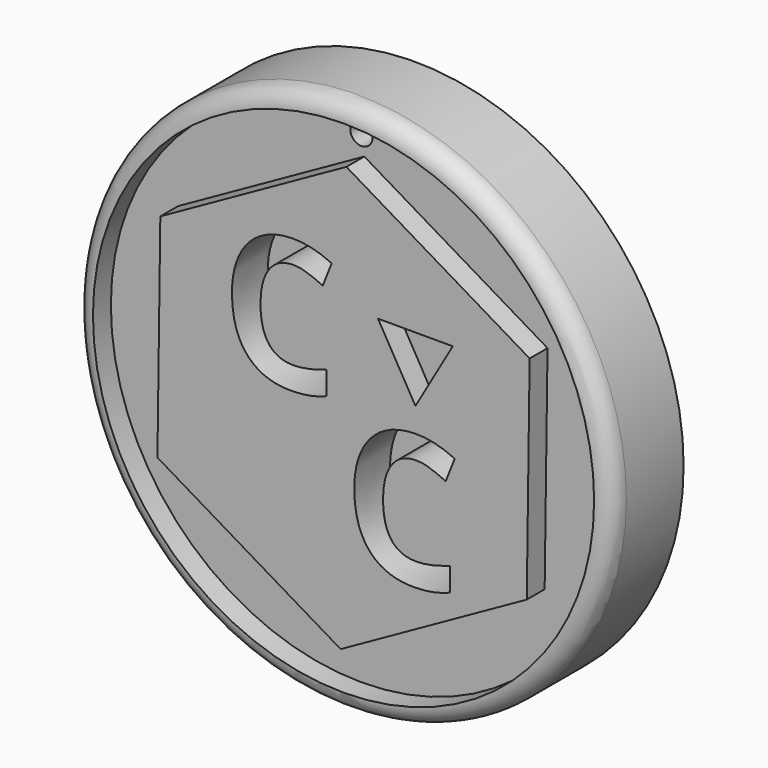
from build123d import *

# Parameters (mm, degrees)
F0_R          = 76.2
F1_DEPTH      = 25.4
F2_R          = 5.08
F5_DEPTH      = 6.35
F3_TEXT_SIZE  = 54.0059381616
F6_DEPTH      = 25.4
F4_TEXT_SIZE  = 39.0783310815
F7_DEPTH      = 25.4
F9_D          = 6.35
F13_DEPTH     = 25.4
F15_DEPTH     = 25.4
F16_DEPTH     = 25.4
F18_DEPTH     = 25.4
F19_DEPTH     = 12.7
F20_TEXT_SIZE = 52.0202641686
F22_DEPTH     = 12.7
F21_TEXT_SIZE = 52.4250945697
F23_DEPTH     = 12.7
F25_DEPTH     = 6.35


# Not quite as in the source:
# - the program builds the solid bodies; features that only make, move or delete a surface that nothing else refers to are left out
# - Text() gives the source's letters only with a copy of the font that has no kerning and outlines rounded to 1/6400 em; it was checked with that copy


with BuildPart() as f1:
    # F0 (on Front) → F1 (new body)
    with BuildSketch(Plane.XZ):
        Circle(F0_R)
    extrude(amount=F1_DEPTH)

    # F2
    f2_edges = [f1.edges().sort_by_distance(p)[0] for p in [
        (-76.2, -25.4, 0),
    ]]
    fillet(f2_edges, radius=F2_R)

    # F5 (cut): a face of the model
    f5_faces = [f1.faces().sort_by_distance(p)[0] for p in [
        (0, -25.4, 0),
    ]]
    extrude(f5_faces, amount=-F5_DEPTH, mode=Mode.SUBTRACT)

    # F3 (on Front) → F6 (join)
    with BuildSketch(Plane.XZ):
        with Locations((-36.0152100115, 0.3191671568)):
            Text('C', F3_TEXT_SIZE, font='Open Sans', font_style=FontStyle.BOLD, text_align=(TextAlign.LEFT, TextAlign.BOTTOM))
    extrude(amount=F6_DEPTH)

    # F4 (on Front) → F7 (join)
    with BuildSketch(Plane.XZ):
        with Locations((0, -30.0425165991)):
            Text('W', F4_TEXT_SIZE, font='Open Sans', font_style=FontStyle.BOLD, text_align=(TextAlign.LEFT, TextAlign.BOTTOM))
    extrude(amount=F7_DEPTH)

    # F9 (through all)
    with Locations(Plane(origin=(0, 0, 0), x_dir=(1, 0, 0), z_dir=(0, 1, 0))):
        with Locations((0, -66.04)):
            Hole(F9_D / 2)

    # F12 (on Front) → F13 (join)
    with BuildSketch(Plane.XZ):
        Polygon((23.8941579933, 39.8077583636), (14.5711407189, 34.4585337912), (10.8677104194, 24.3680700436), (14.5167432909, 14.2578072513), (23.8108162984, 8.858449738), (34.4011293896, 10.6964168913), (41.3323573708, 18.9117034534), (41.3613016377, 29.6602855392), (34.4744188461, 37.9127821335), align=None)
    extrude(amount=F13_DEPTH)

    # F14 (on Front) → F15 (cut)
    with BuildSketch(Plane.XZ):
        Polygon((-48.271715641, 27.8696880196), (-48.271715641, -27.8696880196), (0, -55.7393760392), (48.271715641, -27.8696880196), (48.271715641, 27.8696880196), (0, 55.7393760392), align=None)
    extrude(amount=-F15_DEPTH, mode=Mode.SUBTRACT)

    # F14 (on Front) → F16 (cut)
    with BuildSketch(Plane.XZ):
        Polygon((-48.271715641, 27.8696880196), (-48.271715641, -27.8696880196), (0, -55.7393760392), (48.271715641, -27.8696880196), (48.271715641, 27.8696880196), (0, 55.7393760392), align=None)
    extrude(amount=-F16_DEPTH, mode=Mode.SUBTRACT)

    # F17 (on Front) → F18 (join)
    with BuildSketch(Plane.XZ):
        Polygon((52.8155236149, 29.550879198), (0.8159497178, 60.5150247636), (-51.9995738971, 30.9641455656), (-52.8155236149, -29.550879198), (-0.8159497178, -60.5150247636), (51.9995738971, -30.9641455656), align=None)
    extrude(amount=F18_DEPTH)

    # F17 (on Front) → F19 (cut)
    with BuildSketch(Plane.XZ):
        Polygon((52.8155236149, 29.550879198), (0.8159497178, 60.5150247636), (-51.9995738971, 30.9641455656), (-52.8155236149, -29.550879198), (-0.8159497178, -60.5150247636), (51.9995738971, -30.9641455656), align=None)
    extrude(amount=-F19_DEPTH, mode=Mode.SUBTRACT)

    # F20 (on face) → F22 (cut)
    with BuildSketch(Plane.XZ.offset(25.4)):
        with Locations((-34.6910136674, 0)):
            Text('C', F20_TEXT_SIZE, font='Open Sans', font_style=FontStyle.BOLD, text_align=(TextAlign.LEFT, TextAlign.BOTTOM))
    extrude(amount=-F22_DEPTH, mode=Mode.SUBTRACT)

    # F21 (on face) → F23 (cut)
    with BuildSketch(Plane.XZ.offset(25.4)):
        with Locations((0, -37.7460680902)):
            Text('C', F21_TEXT_SIZE, font='Open Sans', font_style=FontStyle.BOLD, text_align=(TextAlign.LEFT, TextAlign.BOTTOM))
    extrude(amount=-F23_DEPTH, mode=Mode.SUBTRACT)

    # F24 (on face) → F25 (cut)
    with BuildSketch(Plane.XZ.offset(25.4)):
        Polygon((31.0051301991, 25.5040973425), (9.8014277841, 25.5040973425), (20.4032789916, 7.1411523968), align=None)
    extrude(amount=-F25_DEPTH, mode=Mode.SUBTRACT)


solid = f1.part
